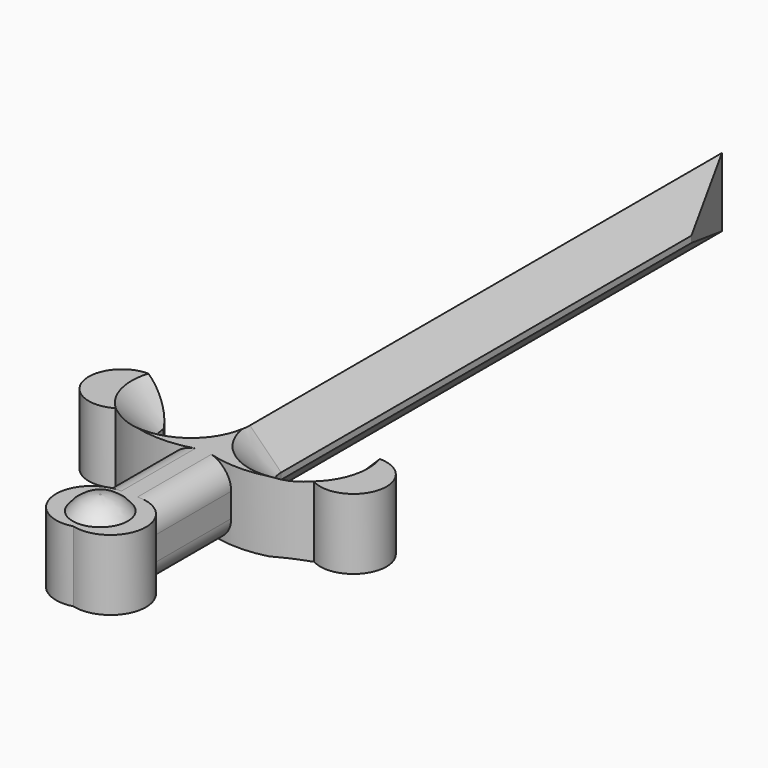
from build123d import *

# Parameters (mm, degrees)
F1_DEPTH     = 11.176
F2_T1_DEPTH  = 94.3857913817
F2_T4_ANGLE  = 351.4780510153
F2_T6_ANGLE  = 351.4780510153
F2_T8_ANGLE  = 351.4780510153
F2_T10_ANGLE = 351.4780510153
F3_R         = 3.6792614691
F4_R         = 3.6792614691
F5_R         = 4.3813050742
F6_DEPTH     = 2.286


# Not quite as in the source:
# - a fillet or chamfer that OpenCascade refuses, or shapes differently, is made with other operations: its cross-section is extruded or revolved along the edge and cut away or added


with BuildPart() as f1:
    # F0 (on Top) → F1 (new body)
    with BuildSketch(Plane.XY):
        with BuildLine():
            Line((4.9550826661, 52.6113137603), (0, 64.8532807827))
            Line((0, 64.8532807827), (-4.9550826661, 52.6113137603))
            Line((-4.9550826661, 52.6113137603), (-4.9550826661, -28.7103280425))
            ThreePointArc((-4.9550826661, -28.7103280425), (-9.3272130471, -33.0824584235), (-13.699343428, -28.7103280425))
            ThreePointArc((-13.699343428, -28.7103280425), (-23.4025628963, -29.6754723169), (-15.7396737486, -35.7057377696))
            ThreePointArc((-15.7396737486, -35.7057377696), (-10.5930074953, -38.0719437204), (-4.9550826661, -38.6204943061))
            Line((-4.9550826661, -38.6204943061), (-4.9550826661, -53.7772104144))
            ThreePointArc((-4.9550826661, -53.7772104144), (-6.5397395867, -60.7633924821), (0, -63.687376678))
            ThreePointArc((0, -63.687376678), (6.5397395867, -60.7633924821), (4.9550826661, -53.7772104144))
            Line((4.9550826661, -53.7772104144), (4.9550826661, -38.6204943061))
            ThreePointArc((4.9550826661, -38.6204943061), (10.5930074953, -38.0719437204), (15.7396737486, -35.7057377696))
            ThreePointArc((15.7396737486, -35.7057377696), (23.4025628963, -29.6754723169), (13.699343428, -28.7103280425))
            ThreePointArc((13.699343428, -28.7103280425), (9.3272130471, -33.0824584235), (4.9550826661, -28.7103280425))
            Line((4.9550826661, -28.7103280425), (4.9550826661, 52.6113137603))
        make_face()
    extrude(amount=F1_DEPTH)

    # F2: chamfer of 5.08 on 8 edges, made by hand

    # F2_s2 → F2_t1 (cut)
    with BuildSketch(Plane.XZ.offset(-65.6754633391)):
        Polygon((-4.9550826661, 6.096), (0.1249173339, 11.176), (-4.9550826661, 11.176), align=None)
        Polygon((4.9550826661, 6.096), (-0.1249173339, 11.176), (4.9550826661, 11.176), align=None)
        Polygon((-4.9550826661, 5.08), (0.1249173339, 0), (-4.9550826661, 0), align=None)
        Polygon((4.9550826661, 5.08), (-0.1249173339, 0), (4.9550826661, 0), align=None)
    extrude(amount=F2_T1_DEPTH, mode=Mode.SUBTRACT)

    # F2_s3 → F2_t4 (revolve, cut)
    with BuildSketch(Plane(origin=(-4.0027369728, -26.7129328444, 0), x_dir=(0, 0, 1), z_dir=(-0.1481882745, -0.9889591677, 0))):
        Polygon((5.08, -9.1066364436), (0, -4.0266364436), (0, -9.1066364436), align=None)
    revolve(axis=Axis((9.3272130471, -28.7103280425, 0), (0, 0, -1)), revolution_arc=F2_T4_ANGLE, mode=Mode.SUBTRACT)

    # F2_s5 → F2_t6 (revolve, cut)
    with BuildSketch(Plane(origin=(-4.0027369728, -26.7129328444, 0), x_dir=(0, 0, 1), z_dir=(-0.1481882745, -0.9889591677, 0))):
        Polygon((6.096, -9.1066364436), (11.176, -4.0266364436), (11.176, -9.1066364436), align=None)
    revolve(axis=Axis((9.3272130471, -28.7103280425, 11.176), (0, 0, -1)), revolution_arc=F2_T6_ANGLE, mode=Mode.SUBTRACT)

    # F2_s7 → F2_t8 (revolve, cut)
    with BuildSketch(Plane.XZ.offset(28.7103280425)):
        Polygon((-4.9550826661, 5.08), (0.1249173339, 0), (-4.9550826661, 0), align=None)
    revolve(axis=Axis((-9.3272130471, -28.7103280425, 0), (0, 0, -1)), revolution_arc=F2_T8_ANGLE, mode=Mode.SUBTRACT)

    # F2_s9 → F2_t10 (revolve, cut)
    with BuildSketch(Plane.XZ.offset(28.7103280425)):
        Polygon((-4.9550826661, 6.096), (0.1249173339, 11.176), (-4.9550826661, 11.176), align=None)
    revolve(axis=Axis((-9.3272130471, -28.7103280425, 11.176), (0, 0, -1)), revolution_arc=F2_T10_ANGLE, mode=Mode.SUBTRACT)

    # F3
    f3_edges = [f1.edges().sort_by_distance(p)[0] for p in [
        (-4.955083, -46.198852, 11.176),
    ]]
    fillet(f3_edges, radius=F3_R)

    # F4
    f4_edges = [f1.edges().sort_by_distance(p)[0] for p in [
        (4.955083, -46.198852, 11.176),
        (4.955083, -46.198852, 0),
        (-4.955083, -46.198852, 0),
    ]]
    fillet(f4_edges, radius=F4_R)

    # F5 (on face) → F6 (join)
    with BuildSketch(Plane.XY.offset(11.176)):
        with Locations((0, -58.3839304745)):
            Circle(F5_R)
    extrude(amount=F6_DEPTH)

    # F7: fillet of radius 5.08 on 1 edges, made by hand

    # F7_s1 → F7_t2 (revolve, cut)
    with BuildSketch(Plane.XZ.offset(58.3839304745)):
        with BuildLine():
            ThreePointArc((4.3813050742, 11.176), (2.5483242068, 12.8541314829), (0.1386686298, 13.462))
            Line((0.1386686298, 13.462), (4.3813050742, 13.462))
            Line((4.3813050742, 13.462), (4.3813050742, 11.176))
        make_face()
    revolve(axis=Axis((0, -58.3839304745, 13.462), (0, 0, 1)), mode=Mode.SUBTRACT)


solid = f1.part
